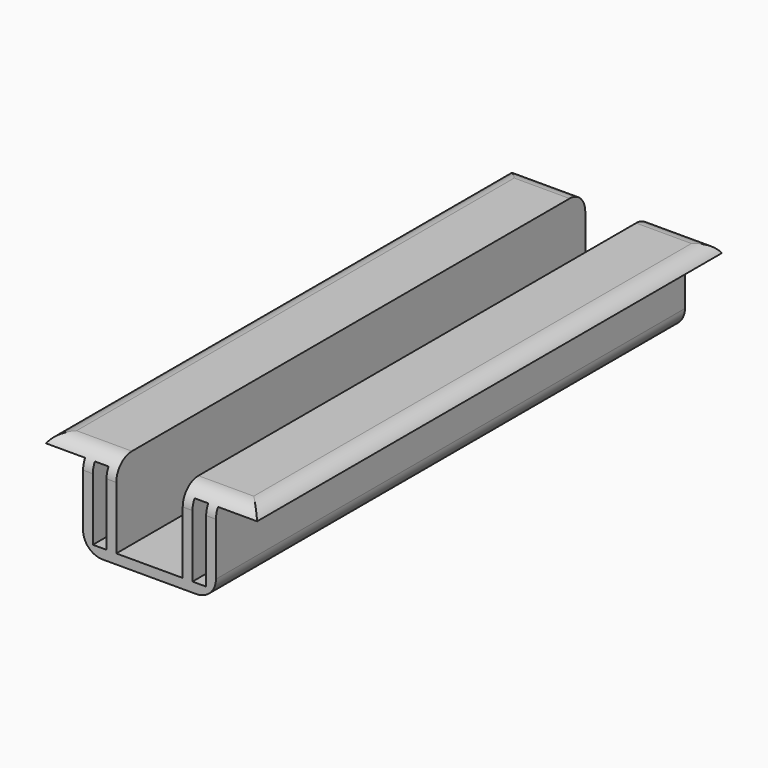
from build123d import *

# Parameters (mm, degrees)
F0_W        = 2.5
F0_H        = 18.5
F1_DEPTH    = 150
F2_T1_DEPTH = 175
F2_T3_DEPTH = 171.6506350946
F2_T5_DEPTH = 43.5
F2_T7_DEPTH = 43.5


# Not quite as in the source:
# - a fillet or chamfer that OpenCascade refuses, or shapes differently, is made with other operations: its cross-section is extruded or revolved along the edge and cut away or added


with BuildPart() as f1:
    # F0 (on Front) → F1 (new body)
    with BuildSketch(Plane.XZ):
        Polygon((-27, 0), (-17, 0), (-14.5, 0), (-14.5, 2.5), (-27, 2.5), align=None)
        Polygon((-11, 0), (-8.5, 0), (-8.5, 2.5), (-14.5, 2.5), (-14.5, 0), align=None)
        with Locations((-9.75, -9.25)):
            Rectangle(F0_W, F0_H)
        with Locations((-15.75, -9.25)):
            Rectangle(F0_W, F0_H)
        Polygon((-17, -21), (0, -21), (0, -18.5), (-8.5, -18.5), (-11, -18.5), (-14.5, -18.5), (-17, -18.5), align=None)
        Polygon((0, -18.5), (0, -21), (17, -21), (17, -18.5), (14.5, -18.5), (11, -18.5), (8.5, -18.5), align=None)
        with Locations((9.75, -9.25)):
            Rectangle(F0_W, F0_H)
        with Locations((15.75, -9.25)):
            Rectangle(F0_W, F0_H)
        Polygon((14.5, 0), (17, 0), (27, 0), (27, 2.5), (14.5, 2.5), align=None)
        Polygon((8.5, 2.5), (8.5, 0), (11, 0), (14.5, 0), (14.5, 2.5), align=None)
    extrude(amount=F1_DEPTH)

    # F2: fillet of radius 5 on 8 edges, made by hand

    # F2_s2 → F2_t1 (cut)
    with BuildSketch(Plane.XZ.offset(-12.5)):
        with BuildLine():
            ThreePointArc((-17, -16), (-15.5355339059, -19.5355339059), (-12, -21))
            Line((-12, -21), (-17, -21))
            Line((-17, -21), (-17, -16))
        make_face()
        with BuildLine():
            ThreePointArc((12, -21), (15.5355339059, -19.5355339059), (17, -16))
            Line((17, -16), (17, -21))
            Line((17, -21), (12, -21))
        make_face()
    extrude(amount=F2_T1_DEPTH, mode=Mode.SUBTRACT)

    # F2_s4 → F2_t3 (cut)
    with BuildSketch(Plane.XZ.offset(-10.8253175473)):
        with BuildLine():
            ThreePointArc((-22.6698729811, 2.5), (-25.1698729811, 1.8301270189), (-27, 0))
            Line((-27, 0), (-27, 2.5))
            Line((-27, 2.5), (-22.6698729811, 2.5))
        make_face()
        with BuildLine():
            ThreePointArc((27, 0), (25.1698729811, 1.8301270189), (22.6698729811, 2.5))
            Line((22.6698729811, 2.5), (27, 2.5))
            Line((27, 2.5), (27, 0))
        make_face()
    extrude(amount=F2_T3_DEPTH, mode=Mode.SUBTRACT)

    # F2_s6 → F2_t5 (cut)
    with BuildSketch(Plane.YZ.offset(-39.5)):
        with BuildLine():
            ThreePointArc((-145, 2.5), (-148.5355339059, 1.0355339059), (-150, -2.5))
            Line((-150, -2.5), (-150, 2.5))
            Line((-150, 2.5), (-145, 2.5))
        make_face()
        with BuildLine():
            ThreePointArc((-5, 2.5), (-1.4644660941, 1.0355339059), (0, -2.5))
            Line((0, -2.5), (0, 2.5))
            Line((0, 2.5), (-5, 2.5))
        make_face()
    extrude(amount=F2_T5_DEPTH, mode=Mode.SUBTRACT)

    # F2_s8 → F2_t7 (cut)
    with BuildSketch(Plane.YZ.offset(-4)):
        with BuildLine():
            ThreePointArc((-145, 2.5), (-148.5355339059, 1.0355339059), (-150, -2.5))
            Line((-150, -2.5), (-150, 2.5))
            Line((-150, 2.5), (-145, 2.5))
        make_face()
        with BuildLine():
            ThreePointArc((-5, 2.5), (-1.4644660941, 1.0355339059), (0, -2.5))
            Line((0, -2.5), (0, 2.5))
            Line((0, 2.5), (-5, 2.5))
        make_face()
    extrude(amount=F2_T7_DEPTH, mode=Mode.SUBTRACT)


solid = f1.part
